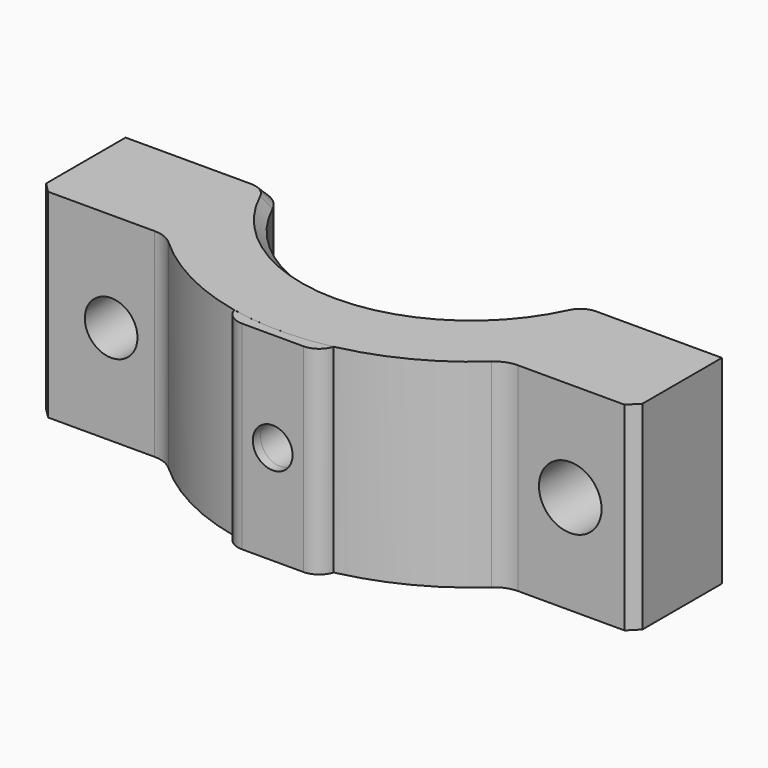
from build123d import *

# Parameters (mm, degrees)
F1_DEPTH     = 20
F2_R         = 3.15
F3_DEPTH     = 6.8
F4_R         = 2.65
F5_DEPTH     = 5.2
F6_R         = 3.15
F7_DEPTH     = 6.8
F8_R         = 2.65
F9_DEPTH     = 5.2
F13_R        = 2
F14_DEPTH    = 30
F15_R        = 3
F16_T1_DEPTH = 29.5768707806
F17_SIZE     = 1


# Not quite as in the source:
# - a fillet or chamfer that OpenCascade refuses, or shapes differently, is made with other operations: its cross-section is extruded or revolved along the edge and cut away or added


with BuildPart() as f1:
    # F0 (on Top) → F1 (new body)
    with BuildSketch(Plane.XY):
        with BuildLine():
            ThreePointArc((15.3039210662, -5), (0, -16.1), (-15.3039210662, -5))
            Line((-15.3039210662, -5), (-30, -5))
            Line((-30, -5), (-30, -17))
            Line((-30, -17), (-17.0824471315, -17))
            ThreePointArc((-17.0824471315, -17), (0, -24.1), (17.0824471315, -17))
            Line((17.0824471315, -17), (30, -17))
            Line((30, -17), (30, -5))
            Line((30, -5), (15.3039210662, -5))
        make_face()
    extrude(amount=F1_DEPTH)

    # F2 (on face) → F3 (cut)
    with BuildSketch(Plane.XZ.offset(17)):
        with Locations((23.5412235657, 10)):
            Circle(F2_R)
    extrude(amount=-F3_DEPTH, mode=Mode.SUBTRACT)

    # F4 (on face) → F5 (cut, through all)
    with BuildSketch(Plane.XZ.offset(10.2)):
        with Locations((23.5412235657, 10)):
            Circle(F4_R)
    extrude(amount=-F5_DEPTH, mode=Mode.SUBTRACT)

    # F6 (on face) → F7 (cut)
    with BuildSketch(Plane(origin=(0, -5, 0), x_dir=(-1, 0, 0), z_dir=(0, 1, 0))):
        with Locations((22.6519605331, 10)):
            Circle(F6_R)
    extrude(amount=-F7_DEPTH, mode=Mode.SUBTRACT)

    # F8 (on face) → F9 (cut, through all)
    with BuildSketch(Plane(origin=(0, -11.8, 0), x_dir=(-1, 0, 0), z_dir=(0, 1, 0))):
        with Locations((22.6519605331, 10)):
            Circle(F8_R)
    extrude(amount=-F9_DEPTH, mode=Mode.SUBTRACT)


with BuildPart() as f12:
    # F11 (on offset) → F12 (new body, up to the next surface of F1)
    with BuildSketch(Plane.XZ.offset(25)):
        Polygon((-5, 0), (0, 0), (5, 0), (5, 20), (-5, 20), align=None)
    extrude(until=Until.NEXT, target=f1.part, dir=(0, 1, 0))


with BuildPart() as f14_tool:
    # F13 (on face) → F14 (new body)
    with BuildSketch(Plane.XZ.offset(25)):
        with Locations((0, 10)):
            Circle(F13_R)
    extrude(amount=-F14_DEPTH)


with BuildPart() as f1_1:
    add(f1.part)

    # F14: cut by f14_tool
    add(f14_tool.part, mode=Mode.SUBTRACT)

    # F15
    f15_edges = [f1_1.edges().sort_by_distance(p)[0] for p in [
        (-15.303921, -5, 10),
        (15.303921, -5, 10),
        (-17.082447, -17, 10),
        (17.082447, -17, 10),
    ]]
    fillet(f15_edges, radius=F15_R)

    # F17
    f17_edges = [f1_1.edges().sort_by_distance(p)[0] for p in [
        (0, -16.1, 0),
        (-23.671937, -5, 20),
        (30, -17, 10),
        (-30, -17, 10),
        (-30, -5, 10),
        (30, -5, 10),
        (0, -16.1, 20),
        (15.726722, -5.473181, 0),
        (-15.726722, -5.473181, 0),
        (23.671937, -5, 0),
        (-23.671937, -5, 0),
        (15.726722, -5.473181, 20),
        (-15.726722, -5.473181, 20),
        (23.671937, -5, 20),
    ]]
    chamfer(f17_edges, length=F17_SIZE)


with BuildPart() as f12_1:
    add(f12.part)

    # F14: cut by f14_tool
    add(f14_tool.part, mode=Mode.SUBTRACT)

    # F16: fillet of radius 2 on 2 edges, made by hand

    # F16_s2 → F16_t1 (cut)
    with BuildSketch(Plane.XY.offset(-4.7884353903)):
        with BuildLine():
            ThreePointArc((-3.0846258439, -25), (-4.2780985066, -24.6048747625), (-5, -23.5756230034))
            Line((-5, -23.5756230034), (-5, -25))
            Line((-5, -25), (-3.0846258439, -25))
        make_face()
        with BuildLine():
            ThreePointArc((3.0846258439, -25), (4.2780985066, -24.6048747625), (5, -23.5756230034))
            Line((5, -23.5756230034), (5, -25))
            Line((5, -25), (3.0846258439, -25))
        make_face()
    extrude(amount=F16_T1_DEPTH, mode=Mode.SUBTRACT)


solid = Compound([f1_1.part, f12_1.part])
